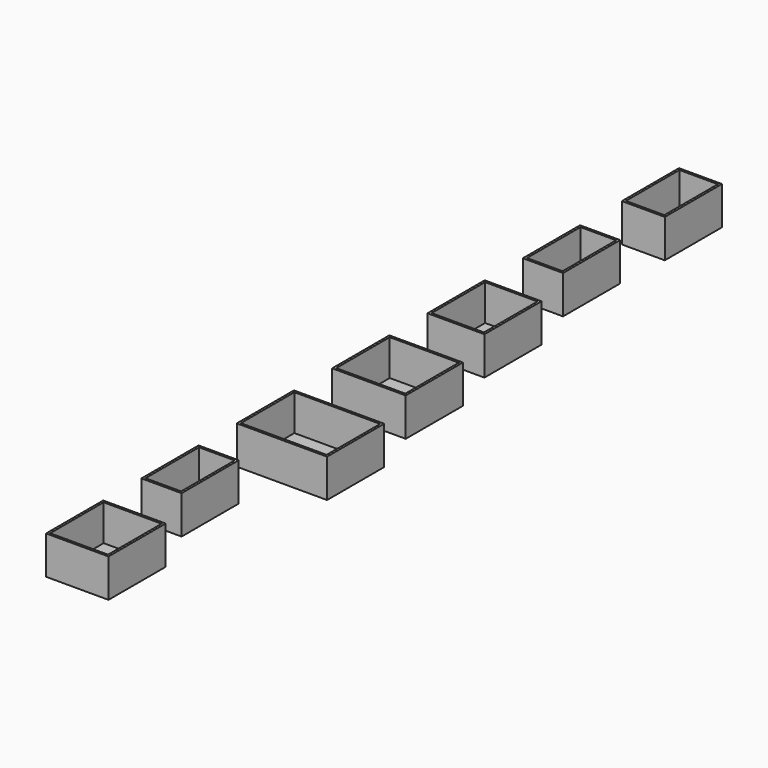
from build123d import *

# Parameters (mm, degrees)
F3_W     = 30.353
F3_H     = 50.4825
F4_DEPTH = 26.9875
F3_W_2   = 28.3845
F3_W_3   = 40.1955
F3_W_4   = 52.0065
F3_W_5   = 63.8175
F3_W_6   = 44.1325
F5_T     = -1.5875
F5_2_T   = -1.5875
F5_3_T   = -1.5875
F5_4_T   = -1.5875
F5_5_T   = -1.5875
F5_6_T   = -1.5875
F5_7_T   = -1.5875


# Not quite as in the source:
# - a variable given as a bare number and used for a length is read in inches; the dataset says mm whatever the document's units were
# - a feature names something its author has since deleted; it is built from what else it names


with BuildPart() as f4:
    # F3 (on Top) → F4 (new body)
    with BuildSketch(Plane.XY):
        with Locations((13.589, 63.7941811943)):
            Rectangle(F3_W, F3_H)
    extrude(amount=F4_DEPTH)

    # F5#7
    f5_7_openings = [f4.faces().sort_by_distance(p)[0] for p in [
        (13.589, 63.794181, 26.9875),
    ]]
    offset(amount=F5_7_T, openings=f5_7_openings)


with BuildPart() as f4b:
    # F3 (on Top) → F4, piece 2 (new body)
    with BuildSketch(Plane.XY):
        with Locations((12.60475, -23.65375)):
            Rectangle(F3_W_2, F3_H)
    extrude(amount=F4_DEPTH)

    # F5#6
    f5_6_openings = [f4b.faces().sort_by_distance(p)[0] for p in [
        (12.60475, -23.65375, 26.9875),
    ]]
    offset(amount=F5_6_T, openings=f5_6_openings)


with BuildPart() as f4c:
    # F3 (on Top) → F4, piece 3 (new body)
    with BuildSketch(Plane.XY):
        with Locations((18.51025, -107.9266811943)):
            Rectangle(F3_W_3, F3_H)
    extrude(amount=F4_DEPTH)

    # F5#5
    f5_5_openings = [f4c.faces().sort_by_distance(p)[0] for p in [
        (18.51025, -107.926681, 26.9875),
    ]]
    offset(amount=F5_5_T, openings=f5_5_openings)


with BuildPart() as f4d:
    # F3 (on Top) → F4, piece 4 (new body)
    with BuildSketch(Plane.XY):
        with Locations((24.41575, -192.1996123886)):
            Rectangle(F3_W_4, F3_H)
    extrude(amount=F4_DEPTH)

    # F5#4
    f5_4_openings = [f4d.faces().sort_by_distance(p)[0] for p in [
        (24.41575, -192.199612, 26.9875),
    ]]
    offset(amount=F5_4_T, openings=f5_4_openings)


with BuildPart() as f4e:
    # F3 (on Top) → F4, piece 5 (new body)
    with BuildSketch(Plane.XY):
        with Locations((30.32125, -276.4725435829)):
            Rectangle(F3_W_5, F3_H)
    extrude(amount=F4_DEPTH)

    # F5#3
    f5_3_openings = [f4e.faces().sort_by_distance(p)[0] for p in [
        (30.32125, -276.472544, 26.9875),
    ]]
    offset(amount=F5_3_T, openings=f5_3_openings)


with BuildPart() as f4f:
    # F3 (on Top) → F4, piece 6 (new body)
    with BuildSketch(Plane.XY):
        with Locations((12.60475, -360.7454747772)):
            Rectangle(F3_W_2, F3_H)
    extrude(amount=F4_DEPTH)

    # F5#2
    f5_2_openings = [f4f.faces().sort_by_distance(p)[0] for p in [
        (12.60475, -360.745475, 26.9875),
    ]]
    offset(amount=F5_2_T, openings=f5_2_openings)


with BuildPart() as f4g:
    # F3 (on Top) → F4, piece 7 (new body)
    with BuildSketch(Plane.XY):
        with Locations((20.47875, -445.0184059715)):
            Rectangle(F3_W_6, F3_H)
    extrude(amount=F4_DEPTH)

    # F5
    f5_openings = [f4g.faces().sort_by_distance(p)[0] for p in [
        (20.47875, -445.018406, 26.9875),
    ]]
    offset(amount=F5_T, openings=f5_openings)


solid = Compound([f4.part, f4b.part, f4c.part, f4d.part, f4e.part, f4f.part, f4g.part])
